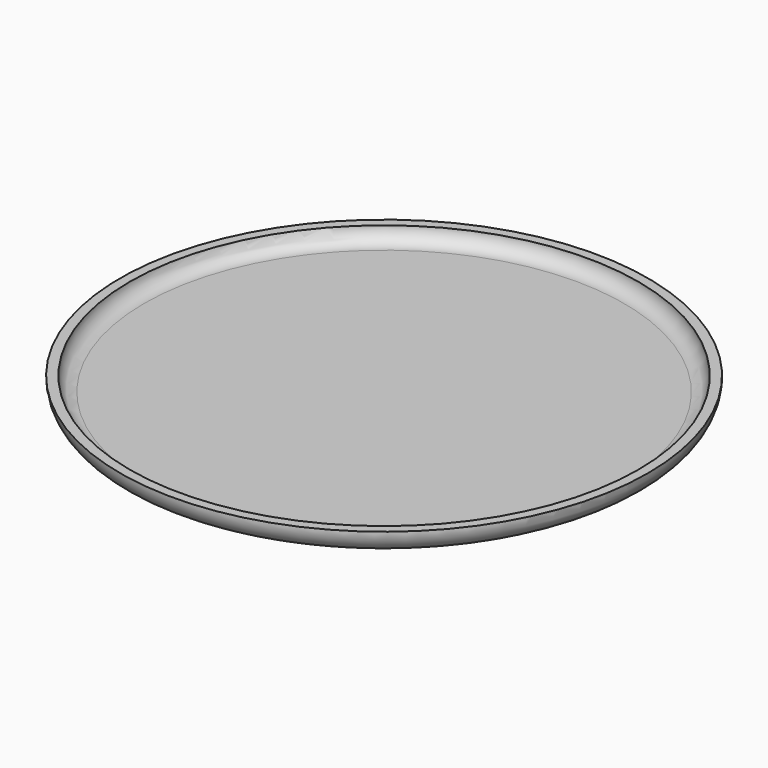
from build123d import *

# Parameters (mm, degrees)
F0_R     = 69.85
F1_DEPTH = 6.35
F2_R     = 6.34999
F3_T     = 2.54


# Not quite as in the source:
# - a fillet or chamfer is up to 0.001 mm smaller than in the source, because OpenCascade refuses the exact size
# - a shell that OpenCascade refuses in one call is made with other operations: the cavity is built on its own and cut out


with BuildPart() as f1:
    # F0 (on Top) → F1 (new body)
    with BuildSketch(Plane.XY):
        Circle(F0_R)
    extrude(amount=F1_DEPTH)

    # F2 (radius 6.35 in the source; OpenCascade refuses exactly that, so slightly less here)
    f2_edges = [f1.edges().sort_by_distance(p)[0] for p in [
        (-69.85, 0, 0),
    ]]
    fillet(f2_edges, radius=F2_R)

    # F3: shell of thickness 2.54, made by hand


with BuildPart() as f3_core1:
    # F3_t2: copy of F1
    add(f1.part)

    # the walls: a layer under each face that stays
    f3_faces = [f3_core1.faces().sort_by_distance(p)[0] for p in [
        (-69.85, 0, 6.349995),
        (-67.9901309895, 0, 1.8598690105),
        (0, 0, 0),
    ]]
    thicken(f3_faces, amount=-F3_T, mode=Mode.SUBTRACT)


with BuildPart() as f1_1:
    add(f1.part)

    # what is left inside the walls is the cavity
    f3_cavity = [f3_core1.part.solids().sort_by_distance(p)[0] for p in [
        (0, -22.436667, 6.3246),
    ]]
    add(f3_cavity, mode=Mode.SUBTRACT)


solid = f1_1.part
